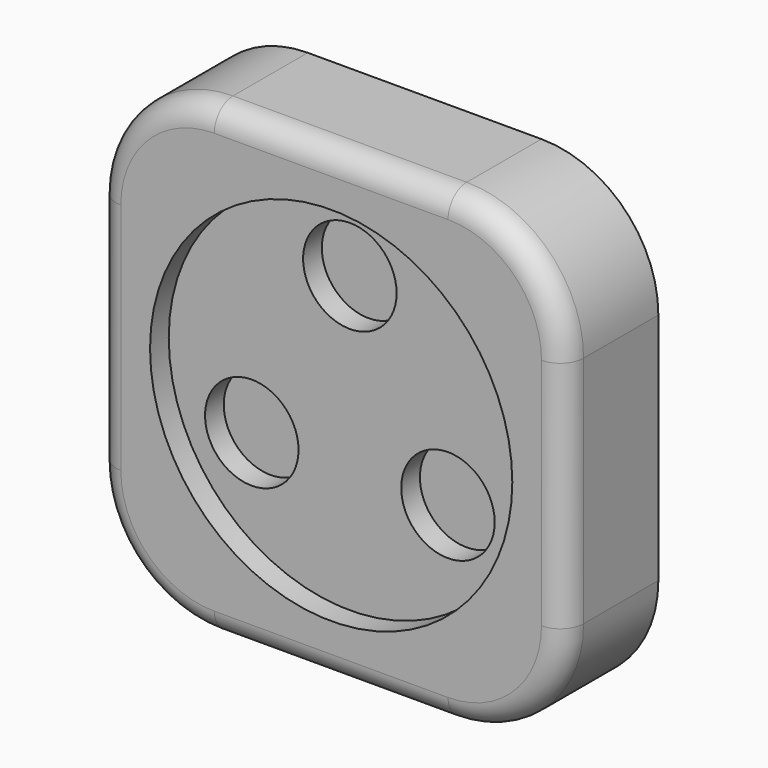
from build123d import *

# Parameters (mm, degrees)
F0_W         = 40
F0_H         = 40
F1_DEPTH     = 10
F2_R         = 15.5
F3_DEPTH     = 2
F4_R         = 4
F5_DEPTH     = 2
F6_R         = 2
F7_T1_DEPTH  = 35
F7_T4_ANGLE  = 90
F7_T6_ANGLE  = 90
F7_T8_ANGLE  = 90
F7_T10_ANGLE = 90


# Not quite as in the source:
# - a fillet or chamfer that OpenCascade refuses, or shapes differently, is made with other operations: its cross-section is extruded or revolved along the edge and cut away or added


with BuildPart() as f1:
    # F0 (on Front) → F1 (new body)
    with BuildSketch(Plane.XZ):
        Rectangle(F0_W, F0_H)
    extrude(amount=F1_DEPTH)

    # F2 (on face) → F3 (cut)
    with BuildSketch(Plane.XZ.offset(10)):
        Circle(F2_R)
    extrude(amount=-F3_DEPTH, mode=Mode.SUBTRACT)

    # F4 (on face) → F5 (cut)
    with BuildSketch(Plane.XZ.offset(8)):
        with Locations((0, 9.6908602864)):
            Circle(F4_R)
        with Locations((-8.3925311925, -4.8454301432)):
            Circle(F4_R)
        with Locations((8.3925311925, -4.8454301432)):
            Circle(F4_R)
    extrude(amount=-F5_DEPTH, mode=Mode.SUBTRACT)

    # F6
    f6_edges = [f1.edges().sort_by_distance(p)[0] for p in [
        (0, -10, 20),
        (-20, -10, 0),
        (20, -10, 0),
        (0, -10, -20),
    ]]
    fillet(f6_edges, radius=F6_R)

    # F7: fillet of radius 10 on 4 edges, made by hand

    # F7_s2 → F7_t1 (cut)
    with BuildSketch(Plane.XZ.offset(-25)):
        with BuildLine():
            ThreePointArc((10, 20), (17.0710678119, 17.0710678119), (20, 10))
            Line((20, 10), (20, 20))
            Line((20, 20), (10, 20))
        make_face()
        with BuildLine():
            ThreePointArc((-10, 20), (-17.0710678119, 17.0710678119), (-20, 10))
            Line((-20, 10), (-20, 20))
            Line((-20, 20), (-10, 20))
        make_face()
        with BuildLine():
            ThreePointArc((20, -10), (17.0710678119, -17.0710678119), (10, -20))
            Line((10, -20), (20, -20))
            Line((20, -20), (20, -10))
        make_face()
        with BuildLine():
            ThreePointArc((-20, -10), (-17.0710678119, -17.0710678119), (-10, -20))
            Line((-10, -20), (-20, -20))
            Line((-20, -20), (-20, -10))
        make_face()
    extrude(amount=F7_T1_DEPTH, mode=Mode.SUBTRACT)

    # F7_s3 → F7_t4 (revolve, cut)
    with BuildSketch(Plane.XY.offset(-10)):
        with BuildLine():
            ThreePointArc((-18, -10), (-19.4142135624, -9.4142135624), (-20, -8))
            Line((-20, -8), (-20, -10))
            Line((-20, -10), (-18, -10))
        make_face()
    revolve(axis=Axis((-10, -10, -10), (0, -1, 0)), revolution_arc=F7_T4_ANGLE, mode=Mode.SUBTRACT)

    # F7_s5 → F7_t6 (revolve, cut)
    with BuildSketch(Plane.YZ.offset(10)):
        with BuildLine():
            ThreePointArc((-10, -18), (-9.4142135624, -19.4142135624), (-8, -20))
            Line((-8, -20), (-10, -20))
            Line((-10, -20), (-10, -18))
        make_face()
    revolve(axis=Axis((10, -10, -10), (0, -1, 0)), revolution_arc=F7_T6_ANGLE, mode=Mode.SUBTRACT)

    # F7_s7 → F7_t8 (revolve, cut)
    with BuildSketch(Plane.YZ.offset(-10)):
        with BuildLine():
            ThreePointArc((-10, 18), (-9.4142135624, 19.4142135624), (-8, 20))
            Line((-8, 20), (-10, 20))
            Line((-10, 20), (-10, 18))
        make_face()
    revolve(axis=Axis((-10, -10, 10), (0, -1, 0)), revolution_arc=F7_T8_ANGLE, mode=Mode.SUBTRACT)

    # F7_s9 → F7_t10 (revolve, cut)
    with BuildSketch(Plane.XY.offset(10)):
        with BuildLine():
            ThreePointArc((18, -10), (19.4142135624, -9.4142135624), (20, -8))
            Line((20, -8), (20, -10))
            Line((20, -10), (18, -10))
        make_face()
    revolve(axis=Axis((10, -10, 10), (0, -1, 0)), revolution_arc=F7_T10_ANGLE, mode=Mode.SUBTRACT)


solid = f1.part
